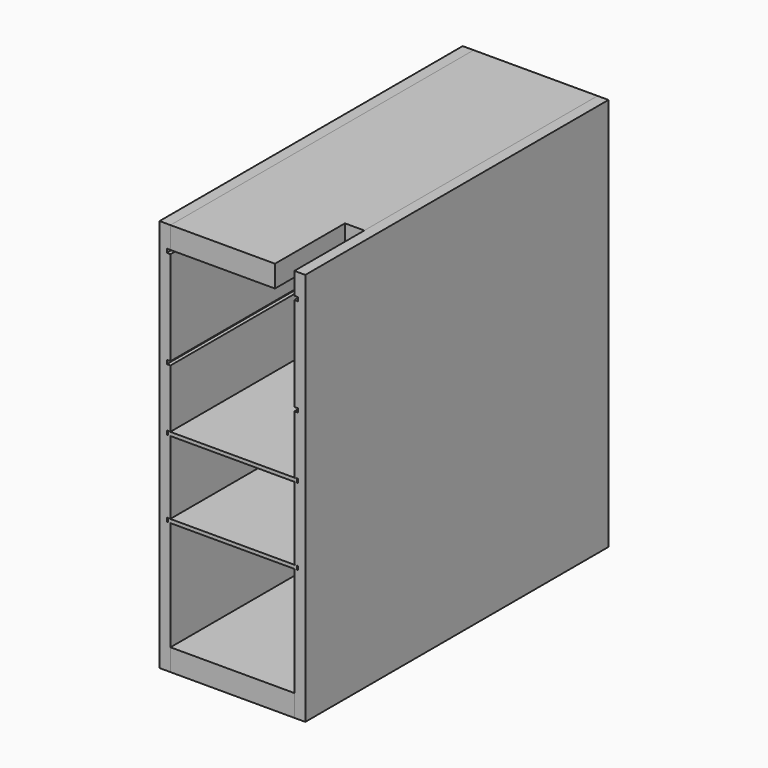
from build123d import *

# Parameters (mm, degrees)
F1_DEPTH  = 330.2
F0_W      = 107.95
F0_H      = 19.05
F2_DEPTH  = 330.2
F3_W      = 112.268
F3_H      = 3.175
F4_DEPTH  = 330.2
F5_W      = 19.05
F5_H      = 25.4
F6_DEPTH  = 3.175
F7_DEPTH  = 225.426
F8_W      = 16.891
F8_H      = 50.8000000001
F9_DEPTH  = 342.901
F10_W     = 112.268
F10_H     = 25.4
F11_DEPTH = 117.476


with BuildPart() as f1:
    # F0 (on Front) → F1 (new body)
    with BuildSketch(Plane.XZ):
        Polygon((0, 342.9), (0, 0), (9.525, 0), (9.525, 19.05), (9.525, 114.3), (6.35, 114.3), (6.35, 117.602), (9.525, 117.602), (9.525, 181.102), (6.35, 181.102), (6.35, 184.404), (9.525, 184.404), (9.525, 235.204), (6.35, 235.204), (6.35, 238.506), (9.525, 238.506), (9.525, 320.548), (6.35, 320.548), (6.35, 323.85), (9.525, 323.85), (9.525, 342.9), align=None)
    extrude(amount=F1_DEPTH)


with BuildPart() as f1b:
    # F0 (on Front) → F1, piece 2 (new body)
    with BuildSketch(Plane.XZ):
        Polygon((117.475, 19.05), (117.475, 0), (127, 0), (127, 342.9), (117.475, 342.9), (117.475, 323.85), (120.65, 323.85), (120.65, 320.548), (117.475, 320.548), (117.475, 238.506), (120.65, 238.506), (120.65, 235.204), (117.475, 235.204), (117.475, 184.404), (120.65, 184.404), (120.65, 181.102), (117.475, 181.102), (117.475, 117.602), (120.65, 117.602), (120.65, 114.3), (117.475, 114.3), align=None)
    extrude(amount=F1_DEPTH)


with BuildPart() as f2:
    # F0 (on Front) → F2 (new body, through all)
    with BuildSketch(Plane.XZ):
        with Locations((63.5, 9.525)):
            Rectangle(F0_W, F0_H)
    extrude(amount=F2_DEPTH)


with BuildPart() as f2b:
    # F0 (on Front) → F2, piece 2 (new body, through all)
    with BuildSketch(Plane.XZ):
        with Locations((63.5, 333.375)):
            Rectangle(F0_W, F0_H)
    extrude(amount=F2_DEPTH)

    # F5 (on face) → F7 (cut, through all)
    with BuildSketch(Plane.XY.offset(117.475)):
        with Locations((110.109, -266.7)):
            Rectangle(F5_W, F5_H)
    extrude(amount=F7_DEPTH, mode=Mode.SUBTRACT)

    # F8 (on face) → F9 (cut, through all)
    with BuildSketch(Plane.XY.offset(342.9)):
        with Locations((109.0295, -304.8000000001)):
            Rectangle(F8_W, F8_H)
    extrude(amount=-F9_DEPTH, mode=Mode.SUBTRACT)


with BuildPart() as f4:
    # F3 (on Front) → F4 (new body, through all)
    with BuildSketch(Plane.XZ):
        with Locations((63.5, 115.8875)):
            Rectangle(F3_W, F3_H)
    extrude(amount=F4_DEPTH)

    # F5 (on face) → F6 (cut, through all)
    with BuildSketch(Plane.XY.offset(117.475)):
        with Locations((110.109, -266.7)):
            Rectangle(F5_W, F5_H)
    extrude(amount=-F6_DEPTH, mode=Mode.SUBTRACT)

    # F10 (on face) → F11 (cut, through all)
    with BuildSketch(Plane.XY.offset(117.475)):
        with Locations((63.5, -12.7)):
            Rectangle(F10_W, F10_H)
    extrude(amount=-F11_DEPTH, mode=Mode.SUBTRACT)


with BuildPart() as f4b:
    # F3 (on Front) → F4, piece 2 (new body, through all)
    with BuildSketch(Plane.XZ):
        with Locations((63.5, 182.6895)):
            Rectangle(F3_W, F3_H)
    extrude(amount=F4_DEPTH)


solid = Compound([f1.part, f1b.part, f2.part, f2b.part, f4.part, f4b.part])
